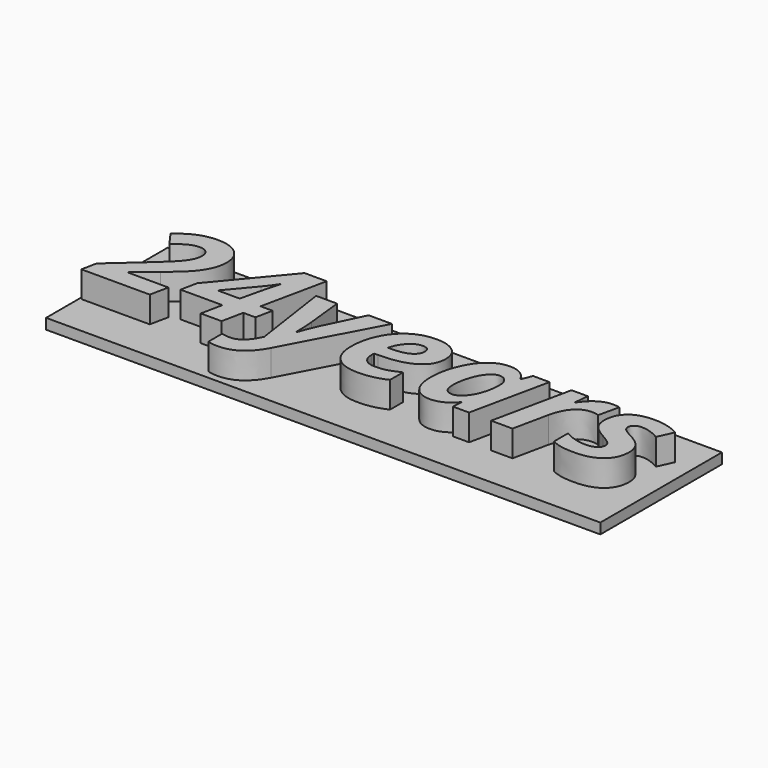
from build123d import *

# Parameters (mm, degrees)
F0_W         = 105.7456597222
F0_H         = 29
F0_TEXT_SIZE = 27.7777777778
F1_DEPTH     = 2
F2_DEPTH     = 5


# Not quite as in the source:
# - a feature names something its author has since deleted; it is built from what else it names
# - Text() gives the source's letters only with a copy of the font that has no kerning and outlines rounded to 1/6400 em; it was checked with that copy


with BuildPart() as f1:
    # F0 (on Top) → F1 (new body)
    with BuildSketch(Plane.XY):
        with Locations((0, 6.5)):
            Rectangle(F0_W, F0_H)
        with BuildLine():
            Line((-17.6671006944, 0), (-19.8893229167, 15.1649305556))
            Line((-19.8893229167, 15.1649305556), (-15.8875868056, 15.1649305556))
            Line((-15.8875868056, 15.1649305556), (-15.1280381944, 8.1380208333))
            add(Edge.make_bspline(
                [(-15.1280381944, 8.1380208333), (-14.94140625, 6.484375), (-14.94140625, 4.1623263889)],
                knots=[0, 0, 0, 1, 1, 1], degree=2))
            Line((-14.94140625, 4.1623263889), (-14.8589409722, 4.1623263889))
            add(Edge.make_bspline(
                [(-14.8589409722, 4.1623263889), (-14.5855034722, 4.8567708333), (-14.2599826389, 5.7855902778)],
                knots=[0, 0, 0, 1, 1, 1], degree=2))
            add(Edge.make_bspline(
                [(-14.2599826389, 5.7855902778), (-13.9344618056, 6.7144097222), (-13.37890625, 7.8689236111)],
                knots=[0, 0, 0, 1, 1, 1], degree=2))
            Line((-13.37890625, 7.8689236111), (-9.8546006944, 15.1649305556))
            Line((-9.8546006944, 15.1649305556), (-5.4188368056, 15.1649305556))
            Line((-5.4188368056, 15.1649305556), (-14.6419270833, -2.1701388889))
            add(Edge.make_bspline(
                [(-14.6419270833, -2.1701388889), (-17.0421006944, -6.6753472222), (-21.19140625, -6.6753472222)],
                knots=[0, 0, 0, 1, 1, 1], degree=2))
            add(Edge.make_bspline(
                [(-21.19140625, -6.6753472222), (-22.4153645833, -6.6753472222), (-23.1879340278, -6.4149305556)],
                knots=[0, 0, 0, 1, 1, 1], degree=2))
            Line((-23.1879340278, -6.4149305556), (-23.1879340278, -3.1597222222))
            add(Edge.make_bspline(
                [(-23.1879340278, -3.1597222222), (-22.2634548611, -3.3376736111), (-21.6124131944, -3.3376736111)],
                knots=[0, 0, 0, 1, 1, 1], degree=2))
            add(Edge.make_bspline(
                [(-21.6124131944, -3.3376736111), (-20.4752604167, -3.3376736111), (-19.6137152778, -2.6866319444)],
                knots=[0, 0, 0, 1, 1, 1], degree=2))
            add(Edge.make_bspline(
                [(-19.6137152778, -2.6866319444), (-18.7521701389, -2.0355902778), (-18.0186631944, -0.6640625)],
                knots=[0, 0, 0, 1, 1, 1], degree=2))
            Line((-18.0186631944, -0.6640625), (-17.6671006944, 0))
        make_face(mode=Mode.SUBTRACT)
        with BuildLine():
            Line((-38.7565104167, 3.5286458333), (-39.4900173611, 0))
            Line((-39.4900173611, 0), (-52.5368923611, 0))
            Line((-52.5368923611, 0), (-51.9552951389, 2.890625))
            Line((-51.9552951389, 2.890625), (-45.4839409722, 8.6414930556))
            add(Edge.make_bspline(
                [(-45.4839409722, 8.6414930556), (-43.0447048611, 10.7986111111), (-42.1137152778, 12.0920138889)],
                knots=[0, 0, 0, 1, 1, 1], degree=2))
            add(Edge.make_bspline(
                [(-42.1137152778, 12.0920138889), (-41.1827256944, 13.3854166667), (-41.1827256944, 14.5269097222)],
                knots=[0, 0, 0, 1, 1, 1], degree=2))
            add(Edge.make_bspline(
                [(-41.1827256944, 14.5269097222), (-41.1827256944, 15.5425347222), (-41.7404513889, 16.0785590278)],
                knots=[0, 0, 0, 1, 1, 1], degree=2))
            add(Edge.make_bspline(
                [(-41.7404513889, 16.0785590278), (-42.2981770833, 16.6145833333), (-43.2313368056, 16.6145833333)],
                knots=[0, 0, 0, 1, 1, 1], degree=2))
            add(Edge.make_bspline(
                [(-43.2313368056, 16.6145833333), (-44.1297743056, 16.6145833333), (-45.0716145833, 16.1610243056)],
                knots=[0, 0, 0, 1, 1, 1], degree=2))
            add(Edge.make_bspline(
                [(-45.0716145833, 16.1610243056), (-46.0134548611, 15.7074652778), (-47.3980034722, 14.5529513889)],
                knots=[0, 0, 0, 1, 1, 1], degree=2))
            Line((-47.3980034722, 14.5529513889), (-49.3771701389, 17.3090277778))
            add(Edge.make_bspline(
                [(-49.3771701389, 17.3090277778), (-47.5846354167, 18.828125), (-45.95703125, 19.4704861111)],
                knots=[0, 0, 0, 1, 1, 1], degree=2))
            add(Edge.make_bspline(
                [(-45.95703125, 19.4704861111), (-44.3294270833, 20.1128472222), (-42.5672743056, 20.1128472222)],
                knots=[0, 0, 0, 1, 1, 1], degree=2))
            add(Edge.make_bspline(
                [(-42.5672743056, 20.1128472222), (-39.9891493056, 20.1128472222), (-38.4852430556, 18.7847222222)],
                knots=[0, 0, 0, 1, 1, 1], degree=2))
            add(Edge.make_bspline(
                [(-38.4852430556, 18.7847222222), (-36.9813368056, 17.4565972222), (-36.9813368056, 15.2734375)],
                knots=[0, 0, 0, 1, 1, 1], degree=2))
            add(Edge.make_bspline(
                [(-36.9813368056, 15.2734375), (-36.9813368056, 13.8194444444), (-37.5368923611, 12.5455729167)],
                knots=[0, 0, 0, 1, 1, 1], degree=2))
            add(Edge.make_bspline(
                [(-37.5368923611, 12.5455729167), (-38.0924479167, 11.2717013889), (-39.1970486111, 9.9956597222)],
                knots=[0, 0, 0, 1, 1, 1], degree=2))
            add(Edge.make_bspline(
                [(-39.1970486111, 9.9956597222), (-40.3016493056, 8.7196180556), (-42.8103298611, 6.6753472222)],
                knots=[0, 0, 0, 1, 1, 1], degree=2))
            Line((-42.8103298611, 6.6753472222), (-46.4605034722, 3.6631944444))
            Line((-46.4605034722, 3.6631944444), (-46.4605034722, 3.5286458333))
            Line((-46.4605034722, 3.5286458333), (-38.7565104167, 3.5286458333))
        make_face(mode=Mode.SUBTRACT)
        Polygon((-21.9379340278, 7.3654513889), (-22.6280381944, 4.1102430556), (-24.9370659722, 4.1102430556), (-25.7921006944, 0), (-29.7634548611, 0), (-28.9084201389, 4.1102430556), (-36.9118923611, 4.1102430556), (-36.2608506944, 7.2829861111), (-25.8181423611, 19.8307291667), (-21.5993923611, 19.8307291667), (-24.2426215278, 7.3654513889), align=None, mode=Mode.SUBTRACT)
        with BuildLine():
            add(Edge.make_bspline(
                [(5.6488715278, 0.8940972222), (3.3181423611, -0.2734375), (0.3624131944, -0.2734375)],
                knots=[0, 0, 0, 1, 1, 1], degree=2))
            add(Edge.make_bspline(
                [(0.3624131944, -0.2734375), (-2.4891493056, -0.2734375), (-4.0625, 1.2608506944)],
                knots=[0, 0, 0, 1, 1, 1], degree=2))
            add(Edge.make_bspline(
                [(-4.0625, 1.2608506944), (-5.6358506944, 2.7951388889), (-5.6358506944, 5.5902777778)],
                knots=[0, 0, 0, 1, 1, 1], degree=2))
            add(Edge.make_bspline(
                [(-5.6358506944, 5.5902777778), (-5.6358506944, 8.3940972222), (-4.5160590278, 10.7074652778)],
                knots=[0, 0, 0, 1, 1, 1], degree=2))
            add(Edge.make_bspline(
                [(-4.5160590278, 10.7074652778), (-3.3962673611, 13.0208333333), (-1.484375, 14.2339409722)],
                knots=[0, 0, 0, 1, 1, 1], degree=2))
            add(Edge.make_bspline(
                [(-1.484375, 14.2339409722), (0.4275173611, 15.4470486111), (2.8407118056, 15.4470486111)],
                knots=[0, 0, 0, 1, 1, 1], degree=2))
            add(Edge.make_bspline(
                [(2.8407118056, 15.4470486111), (5.2452256944, 15.4470486111), (6.5863715278, 14.3424479167)],
                knots=[0, 0, 0, 1, 1, 1], degree=2))
            add(Edge.make_bspline(
                [(6.5863715278, 14.3424479167), (7.9275173611, 13.2378472222), (7.9275173611, 11.3107638889)],
                knots=[0, 0, 0, 1, 1, 1], degree=2))
            add(Edge.make_bspline(
                [(7.9275173611, 11.3107638889), (7.9275173611, 8.7760416667), (5.6640625, 7.4001736111)],
                knots=[0, 0, 0, 1, 1, 1], degree=2))
            add(Edge.make_bspline(
                [(5.6640625, 7.4001736111), (3.4006076389, 6.0243055556), (-0.8051215278, 6.0243055556)],
                knots=[0, 0, 0, 1, 1, 1], degree=2))
            Line((-0.8051215278, 6.0243055556), (-1.4995659722, 6.0243055556))
            Line((-1.4995659722, 6.0243055556), (-1.5256076389, 5.7378472222))
            Line((-1.5256076389, 5.7378472222), (-1.5256076389, 5.4644097222))
            add(Edge.make_bspline(
                [(-1.5256076389, 5.4644097222), (-1.5256076389, 4.2317708333), (-0.8268229167, 3.5199652778)],
                knots=[0, 0, 0, 1, 1, 1], degree=2))
            add(Edge.make_bspline(
                [(-0.8268229167, 3.5199652778), (-0.1280381944, 2.8081597222), (1.1740451389, 2.8081597222)],
                knots=[0, 0, 0, 1, 1, 1], degree=2))
            add(Edge.make_bspline(
                [(1.1740451389, 2.8081597222), (2.3546006944, 2.8081597222), (3.3181423611, 3.06640625)],
                knots=[0, 0, 0, 1, 1, 1], degree=2))
            add(Edge.make_bspline(
                [(3.3181423611, 3.06640625), (4.2816840278, 3.3246527778), (5.6488715278, 3.9756944444)],
                knots=[0, 0, 0, 1, 1, 1], degree=2))
            Line((5.6488715278, 3.9756944444), (5.6488715278, 0.8940972222))
        make_face(mode=Mode.SUBTRACT)
        with BuildLine():
            add(Edge.make_bspline(
                [(18.45703125, 1.9661458333), (16.6384548611, -0.2734375), (14.1297743056, -0.2734375)],
                knots=[0, 0, 0, 1, 1, 1], degree=2))
            add(Edge.make_bspline(
                [(14.1297743056, -0.2734375), (12.1332465278, -0.2734375), (10.9874131944, 1.171875)],
                knots=[0, 0, 0, 1, 1, 1], degree=2))
            add(Edge.make_bspline(
                [(10.9874131944, 1.171875), (9.8415798611, 2.6171875), (9.8415798611, 5.2213541667)],
                knots=[0, 0, 0, 1, 1, 1], degree=2))
            add(Edge.make_bspline(
                [(9.8415798611, 5.2213541667), (9.8415798611, 7.9079861111), (10.8181423611, 10.3428819444)],
                knots=[0, 0, 0, 1, 1, 1], degree=2))
            add(Edge.make_bspline(
                [(10.8181423611, 10.3428819444), (11.7947048611, 12.7777777778), (13.3832465278, 14.1124131944)],
                knots=[0, 0, 0, 1, 1, 1], degree=2))
            add(Edge.make_bspline(
                [(13.3832465278, 14.1124131944), (14.9717881944, 15.4470486111), (16.8684895833, 15.4470486111)],
                knots=[0, 0, 0, 1, 1, 1], degree=2))
            add(Edge.make_bspline(
                [(16.8684895833, 15.4470486111), (18.18359375, 15.4470486111), (19.140625, 14.8784722222)],
                knots=[0, 0, 0, 1, 1, 1], degree=2))
            add(Edge.make_bspline(
                [(19.140625, 14.8784722222), (20.09765625, 14.3098958333), (20.6271701389, 13.2248263889)],
                knots=[0, 0, 0, 1, 1, 1], degree=2))
            Line((20.6271701389, 13.2248263889), (20.7356770833, 13.2248263889))
            Line((20.7356770833, 13.2248263889), (21.5082465278, 15.1649305556))
            Line((21.5082465278, 15.1649305556), (24.6549479167, 15.1649305556))
            Line((24.6549479167, 15.1649305556), (21.42578125, 0))
            Line((21.42578125, 0), (18.3181423611, 0))
            Line((18.3181423611, 0), (18.5091145833, 1.9661458333))
            Line((18.5091145833, 1.9661458333), (18.45703125, 1.9661458333))
        make_face(mode=Mode.SUBTRACT)
        with BuildLine():
            add(Edge.make_bspline(
                [(31.7599826389, 12.3567708333), (33.7565104167, 15.4470486111), (36.5473090278, 15.4470486111)],
                knots=[0, 0, 0, 1, 1, 1], degree=2))
            add(Edge.make_bspline(
                [(36.5473090278, 15.4470486111), (37.3502604167, 15.4470486111), (37.8493923611, 15.2994791667)],
                knots=[0, 0, 0, 1, 1, 1], degree=2))
            Line((37.8493923611, 15.2994791667), (36.9552951389, 11.3671875))
            add(Edge.make_bspline(
                [(36.9552951389, 11.3671875), (36.3433159722, 11.5842013889), (35.6011284722, 11.5842013889)],
                knots=[0, 0, 0, 1, 1, 1], degree=2))
            add(Edge.make_bspline(
                [(35.6011284722, 11.5842013889), (34.0256076389, 11.5842013889), (32.8385416667, 10.3428819444)],
                knots=[0, 0, 0, 1, 1, 1], degree=2))
            add(Edge.make_bspline(
                [(32.8385416667, 10.3428819444), (31.6514756944, 9.1015625), (31.15234375, 6.7838541667)],
                knots=[0, 0, 0, 1, 1, 1], degree=2))
            Line((31.15234375, 6.7838541667), (29.7113715278, 0))
            Line((29.7113715278, 0), (25.6315104167, 0))
            Line((25.6315104167, 0), (28.8433159722, 15.1649305556))
            Line((28.8433159722, 15.1649305556), (31.9639756944, 15.1649305556))
            Line((31.9639756944, 15.1649305556), (31.6775173611, 12.3567708333))
            Line((31.6775173611, 12.3567708333), (31.7599826389, 12.3567708333))
        make_face(mode=Mode.SUBTRACT)
        with BuildLine():
            add(Edge.make_bspline(
                [(47.3198784722, 7.3111979167), (48.06640625, 6.3064236111), (48.06640625, 5.0043402778)],
                knots=[0, 0, 0, 1, 1, 1], degree=2))
            add(Edge.make_bspline(
                [(48.06640625, 5.0043402778), (48.06640625, 2.4565972222), (46.3780381944, 1.0915798611)],
                knots=[0, 0, 0, 1, 1, 1], degree=2))
            add(Edge.make_bspline(
                [(46.3780381944, 1.0915798611), (44.6896701389, -0.2734375), (41.6775173611, -0.2734375)],
                knots=[0, 0, 0, 1, 1, 1], degree=2))
            add(Edge.make_bspline(
                [(41.6775173611, -0.2734375), (40.2235243056, -0.2734375), (39.1471354167, -0.0694444444)],
                knots=[0, 0, 0, 1, 1, 1], degree=2))
            add(Edge.make_bspline(
                [(39.1471354167, -0.0694444444), (38.0707465278, 0.1345486111), (37.1332465278, 0.6119791667)],
                knots=[0, 0, 0, 1, 1, 1], degree=2))
            Line((37.1332465278, 0.6119791667), (37.1332465278, 3.9756944444))
            add(Edge.make_bspline(
                [(37.1332465278, 3.9756944444), (39.2643229167, 2.7517361111), (41.4605034722, 2.7517361111)],
                knots=[0, 0, 0, 1, 1, 1], degree=2))
            add(Edge.make_bspline(
                [(41.4605034722, 2.7517361111), (42.5455729167, 2.7517361111), (43.2378472222, 3.1944444444)],
                knots=[0, 0, 0, 1, 1, 1], degree=2))
            add(Edge.make_bspline(
                [(43.2378472222, 3.1944444444), (43.9301215278, 3.6371527778), (43.9301215278, 4.3967013889)],
                knots=[0, 0, 0, 1, 1, 1], degree=2))
            add(Edge.make_bspline(
                [(43.9301215278, 4.3967013889), (43.9301215278, 4.9782986111), (43.4266493056, 5.4383680556)],
                knots=[0, 0, 0, 1, 1, 1], degree=2))
            add(Edge.make_bspline(
                [(43.4266493056, 5.4383680556), (42.9231770833, 5.8984375), (41.6514756944, 6.6059027778)],
                knots=[0, 0, 0, 1, 1, 1], degree=2))
            add(Edge.make_bspline(
                [(41.6514756944, 6.6059027778), (40.0065104167, 7.5260416667), (39.35546875, 8.4418402778)],
                knots=[0, 0, 0, 1, 1, 1], degree=2))
            add(Edge.make_bspline(
                [(39.35546875, 8.4418402778), (38.7044270833, 9.3576388889), (38.7044270833, 10.6076388889)],
                knots=[0, 0, 0, 1, 1, 1], degree=2))
            add(Edge.make_bspline(
                [(38.7044270833, 10.6076388889), (38.7044270833, 12.9123263889), (40.2039930556, 14.1796875)],
                knots=[0, 0, 0, 1, 1, 1], degree=2))
            add(Edge.make_bspline(
                [(40.2039930556, 14.1796875), (41.7035590278, 15.4470486111), (44.4856770833, 15.4470486111)],
                knots=[0, 0, 0, 1, 1, 1], degree=2))
            add(Edge.make_bspline(
                [(44.4856770833, 15.4470486111), (47.2113715278, 15.4470486111), (49.4075520833, 14.1623263889)],
                knots=[0, 0, 0, 1, 1, 1], degree=2))
            Line((49.4075520833, 14.1623263889), (48.06640625, 11.2456597222))
            add(Edge.make_bspline(
                [(48.06640625, 11.2456597222), (46.1653645833, 12.3828125), (44.5638020833, 12.3828125)],
                knots=[0, 0, 0, 1, 1, 1], degree=2))
            add(Edge.make_bspline(
                [(44.5638020833, 12.3828125), (43.7912326389, 12.3828125), (43.3181423611, 12.0377604167)],
                knots=[0, 0, 0, 1, 1, 1], degree=2))
            add(Edge.make_bspline(
                [(43.3181423611, 12.0377604167), (42.8450520833, 11.6927083333), (42.8450520833, 11.1067708333)],
                knots=[0, 0, 0, 1, 1, 1], degree=2))
            add(Edge.make_bspline(
                [(42.8450520833, 11.1067708333), (42.8450520833, 10.5815972222), (43.2790798611, 10.1801215278)],
                knots=[0, 0, 0, 1, 1, 1], degree=2))
            add(Edge.make_bspline(
                [(43.2790798611, 10.1801215278), (43.7131076389, 9.7786458333), (44.9066840278, 9.1710069444)],
                knots=[0, 0, 0, 1, 1, 1], degree=2))
            add(Edge.make_bspline(
                [(44.9066840278, 9.1710069444), (46.5733506944, 8.3159722222), (47.3198784722, 7.3111979167)],
                knots=[0, 0, 0, 1, 1, 1], degree=2))
        make_face(mode=Mode.SUBTRACT)
        with Locations((-51.8728298611, 0)):
            Text('24years', F0_TEXT_SIZE, font='Open Sans', font_style=FontStyle.BOLDITALIC, text_align=(TextAlign.LEFT, TextAlign.BOTTOM))
        with BuildLine():
            add(Edge.make_bspline(
                [(14.43359375, 3.6219618056), (14.8893229167, 3.0251736111), (15.7313368056, 3.0251736111)],
                knots=[0, 0, 0, 1, 1, 1], degree=2))
            add(Edge.make_bspline(
                [(15.7313368056, 3.0251736111), (16.6644965278, 3.0251736111), (17.5325520833, 3.9344618056)],
                knots=[0, 0, 0, 1, 1, 1], degree=2))
            add(Edge.make_bspline(
                [(17.5325520833, 3.9344618056), (18.4006076389, 4.84375), (18.9301215278, 6.3953993056)],
                knots=[0, 0, 0, 1, 1, 1], degree=2))
            add(Edge.make_bspline(
                [(18.9301215278, 6.3953993056), (19.4596354167, 7.9470486111), (19.4596354167, 9.9131944444)],
                knots=[0, 0, 0, 1, 1, 1], degree=2))
            add(Edge.make_bspline(
                [(19.4596354167, 9.9131944444), (19.4596354167, 10.8767361111), (18.9366319444, 11.5082465278)],
                knots=[0, 0, 0, 1, 1, 1], degree=2))
            add(Edge.make_bspline(
                [(18.9366319444, 11.5082465278), (18.4136284722, 12.1397569444), (17.55859375, 12.1397569444)],
                knots=[0, 0, 0, 1, 1, 1], degree=2))
            add(Edge.make_bspline(
                [(17.55859375, 12.1397569444), (16.6384548611, 12.1397569444), (15.8051215278, 11.1631944444)],
                knots=[0, 0, 0, 1, 1, 1], degree=2))
            add(Edge.make_bspline(
                [(15.8051215278, 11.1631944444), (14.9717881944, 10.1866319444), (14.4748263889, 8.5850694444)],
                knots=[0, 0, 0, 1, 1, 1], degree=2))
            add(Edge.make_bspline(
                [(14.4748263889, 8.5850694444), (13.9778645833, 6.9835069444), (13.9778645833, 5.4123263889)],
                knots=[0, 0, 0, 1, 1, 1], degree=2))
            add(Edge.make_bspline(
                [(13.9778645833, 5.4123263889), (13.9778645833, 4.21875), (14.43359375, 3.6219618056)],
                knots=[0, 0, 0, 1, 1, 1], degree=2))
        make_face()
        with BuildLine():
            Line((-32.4370659722, 7.3654513889), (-28.2183159722, 7.3654513889))
            Line((-28.2183159722, 7.3654513889), (-27.4327256944, 10.7291666667))
            add(Edge.make_bspline(
                [(-27.4327256944, 10.7291666667), (-27.2677951389, 11.5147569444), (-26.8880208333, 12.9535590278)],
                knots=[0, 0, 0, 1, 1, 1], degree=2))
            add(Edge.make_bspline(
                [(-26.8880208333, 12.9535590278), (-26.5082465278, 14.3923611111), (-26.3172743056, 14.8654513889)],
                knots=[0, 0, 0, 1, 1, 1], degree=2))
            Line((-26.3172743056, 14.8654513889), (-26.3997395833, 14.8654513889))
            add(Edge.make_bspline(
                [(-26.3997395833, 14.8654513889), (-26.8771701389, 14.0104166667), (-28.1922743056, 12.4088541667)],
                knots=[0, 0, 0, 1, 1, 1], degree=2))
            Line((-28.1922743056, 12.4088541667), (-32.4370659722, 7.3654513889))
        make_face()
        with BuildLine():
            add(Edge.make_bspline(
                [(4.0082465278, 11.2152777778), (4.0082465278, 12.5043402778), (2.5846354167, 12.5043402778)],
                knots=[0, 0, 0, 1, 1, 1], degree=2))
            add(Edge.make_bspline(
                [(2.5846354167, 12.5043402778), (1.3910590278, 12.5043402778), (0.3342013889, 11.4192708333)],
                knots=[0, 0, 0, 1, 1, 1], degree=2))
            add(Edge.make_bspline(
                [(0.3342013889, 11.4192708333), (-0.72265625, 10.3342013889), (-1.0481770833, 8.7760416667)],
                knots=[0, 0, 0, 1, 1, 1], degree=2))
            Line((-1.0481770833, 8.7760416667), (-0.4405381944, 8.7760416667))
            add(Edge.make_bspline(
                [(-0.4405381944, 8.7760416667), (1.6644965278, 8.7760416667), (2.8363715278, 9.43359375)],
                knots=[0, 0, 0, 1, 1, 1], degree=2))
            add(Edge.make_bspline(
                [(2.8363715278, 9.43359375), (4.0082465278, 10.0911458333), (4.0082465278, 11.2152777778)],
                knots=[0, 0, 0, 1, 1, 1], degree=2))
        make_face()
    extrude(amount=-F1_DEPTH)

    # F0 (on Top) → F2 (join)
    with BuildSketch(Plane.XY):
        with Locations((-51.8728298611, 0)):
            Text('24years', F0_TEXT_SIZE, font='Open Sans', font_style=FontStyle.BOLDITALIC, text_align=(TextAlign.LEFT, TextAlign.BOTTOM))
    extrude(amount=F2_DEPTH)


solid = f1.part
